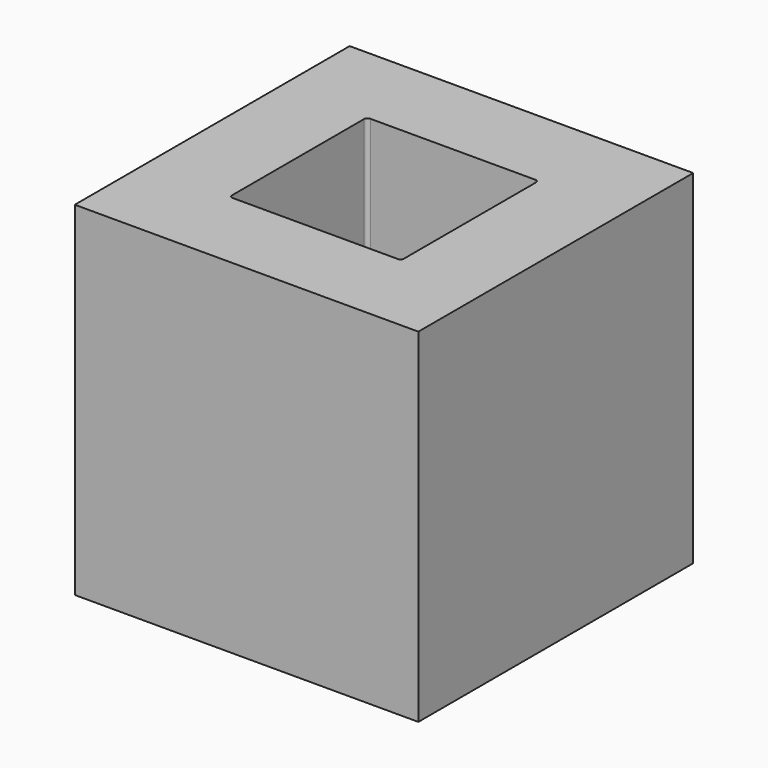
from build123d import *

# Parameters (mm, degrees)
F0_W     = 101.6
F0_H     = 101.6
F1_DEPTH = 50.8
F2_W     = 50.8
F2_H     = 50.8
F3_DEPTH = 50.8
F4_R     = 1.016


with BuildPart() as f1:
    # F0 (on Front) → F1 (new body, symmetric)
    with BuildSketch(Plane.XZ):
        Rectangle(F0_W, F0_H)
    extrude(amount=F1_DEPTH, both=True)

    # F2 (on Top) → F3 (cut, symmetric)
    with BuildSketch(Plane.XY):
        Rectangle(F2_W, F2_H)
    extrude(amount=F3_DEPTH, both=True, mode=Mode.SUBTRACT)

    # F4
    f4_edges = [f1.edges().sort_by_distance(p)[0] for p in [
        (-25.4, -25.4, 0),
        (-25.4, 25.4, 0),
        (25.4, 25.4, 0),
        (25.4, -25.4, 0),
    ]]
    fillet(f4_edges, radius=F4_R)


solid = f1.part
